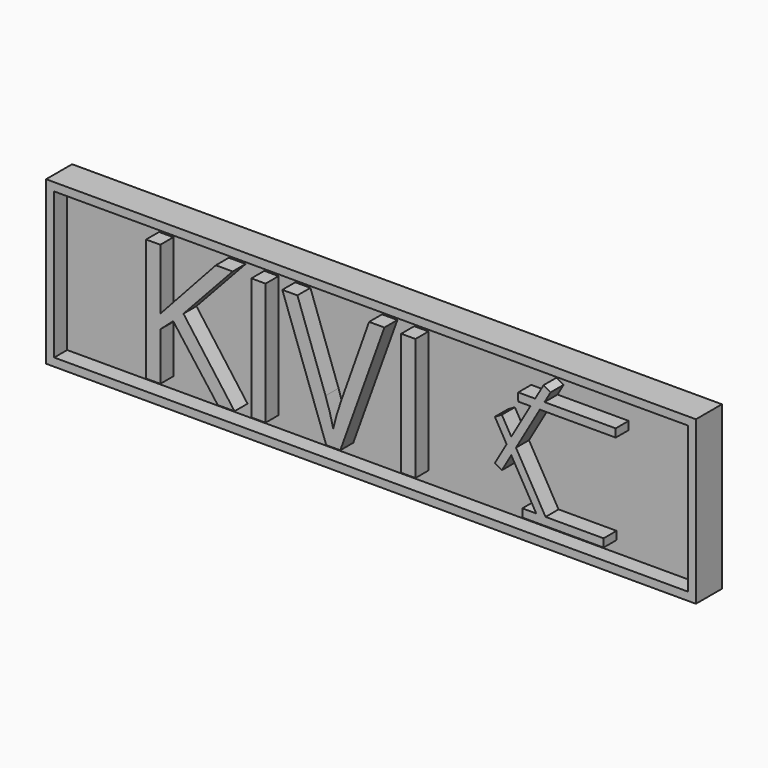
from build123d import *

# Parameters (mm, degrees)
F3_DEPTH     = 2
F0_W         = 0.5
F0_H         = 9
F0_W_2       = 39
F0_H_2       = 0.5
F1_TEXT_SIZE = 10.5555555556
F4_DEPTH     = 2
F5_DEPTH     = 1
F6_DEPTH     = 2


# Not quite as in the source:
# - a feature names something its author has since deleted; it is built from what else it names
# - Text() gives the source's letters only with a copy of the font that has no kerning and outlines rounded to 1/6400 em; it was checked with that copy


with BuildPart() as f3:
    # F2 (on face) → F3 (new body)
    with BuildSketch(Plane.XZ):
        Polygon((9.0606113665, 2.9), (9.0639101416, 2.400010882), (9.8144654915, 2.400010882), (10.1031343434, 2.9), align=None)
        Polygon((10.1031343434, 2.9), (9.8144654915, 2.400010882), (10.3918157607, 2.400010882), (10.6804846126, 2.9), align=None)
        Polygon((10.3918157607, 2.400010882), (9.8144654915, 2.400010882), (8.6348446075, 0.3568475773), (8.9235197421, -0.1431524227), align=None)
        Polygon((10.6804846126, 2.9), (10.3918157607, 2.400010882), (15.0639101416, 2.400010882), (15.0606113665, 2.9), align=None)
        Polygon((8.9235197421, -0.1431524227), (8.6348446075, 0.3568475773), (8.346169473, -0.1431524227), (8.6348446075, -0.6431524227), align=None)
        Polygon((8.346169473, -0.1431524227), (8.6348446075, 0.3568475773), (8.0555336327, 1.3602436191), (7.6225209308, 1.1102436191), align=None)
        Polygon((10.6227495857, 3.8), (10.1031343434, 2.9), (10.6804846126, 2.9), (11.0557622876, 3.55), align=None)
        Polygon((10.7461265406, -3.2999999998), (8.9235197421, -0.1431524227), (8.6348446075, -0.6431524227), (10.1687762714, -3.2999999999), align=None)
        Polygon((8.6348446075, -0.6431524227), (8.346169473, -0.1431524227), (7.6227495857, -1.3961524227), (8.0557622876, -1.6461524227), align=None)
        Polygon((14.3165753115, -3.2999999993), (10.7461265406, -3.2999999998), (10.8055336327, -3.4028961017), (10.3725209308, -3.6528961017), (10.1687762714, -3.2999999999), (9.3165753115, -3.3), (9.3165753182, -3.8), (14.3165753182, -3.7999999993), align=None)
        Polygon((10.8055336327, -3.4028961017), (10.7461265406, -3.2999999998), (10.1687762714, -3.2999999999), (10.3725209308, -3.6528961017), align=None)
    extrude(amount=F3_DEPTH)


with BuildPart() as f3b:
    # F0 (on Front) → F3, piece 2 (new body)
    with BuildSketch(Plane.XZ):
        Polygon((19.5, 5), (-20, 5), (-20, 4.5), (-19.5, 4.5), (19.5, 4.5), align=None)
        with Locations((-19.75, 0)):
            Rectangle(F0_W, F0_H)
        with Locations((0, -4.75)):
            Rectangle(F0_W_2, F0_H_2)
        with Locations((-19.75, -4.75)):
            Rectangle(F0_W, F0_H_2)
        with Locations((19.75, -4.75)):
            Rectangle(F0_W, F0_H_2)
        with Locations((19.75, 0)):
            Rectangle(F0_W, F0_H)
        with Locations((19.75, 4.75)):
            Rectangle(F0_W, F0_H_2)
    extrude(amount=F3_DEPTH)


with BuildPart() as f4:
    # F1 (on face) → F4 (new body)
    with BuildSketch(Plane.XZ):
        with Locations((-14.8792501899, -3.8)):
            Text('KIVI', F1_TEXT_SIZE, font='Open Sans', text_align=(TextAlign.LEFT, TextAlign.BOTTOM))
    extrude(amount=F4_DEPTH)

    # F1 (on face) → F6 (join)
    with BuildSketch(Plane.XZ):
        with Locations((-14.8792501899, -3.8)):
            Text('KIVI', F1_TEXT_SIZE, font='Open Sans', text_align=(TextAlign.LEFT, TextAlign.BOTTOM))
    extrude(amount=F6_DEPTH)


with BuildPart() as f5:
    # F0 (on Front) → F5 (new body)
    with BuildSketch(Plane.XZ):
        Rectangle(F0_W_2, F0_H)
    extrude(amount=F5_DEPTH)


solid = Compound([f3.part, f3b.part, f4.part, f5.part])
